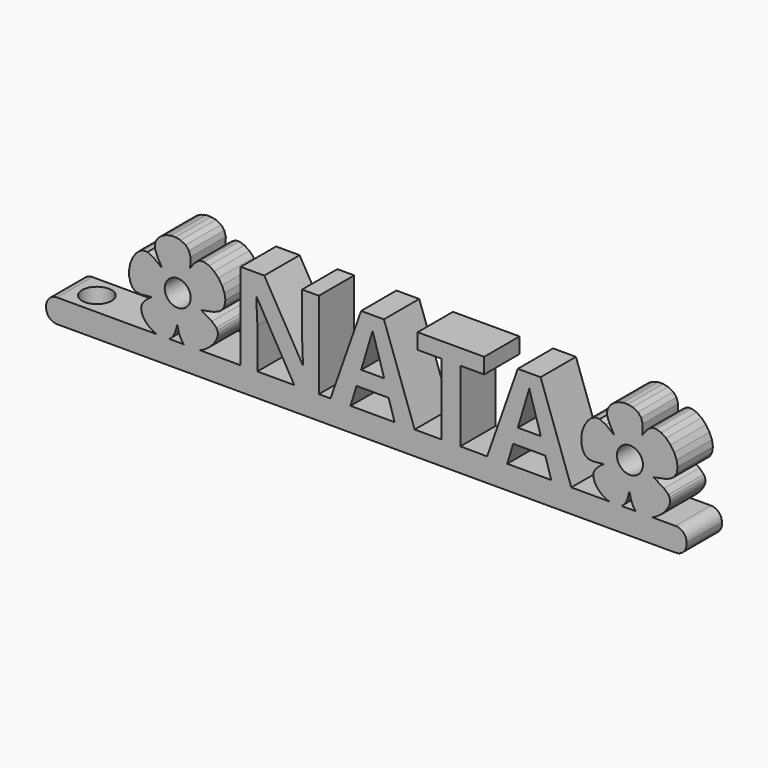
from build123d import *

# Parameters (mm, degrees)
F0_R         = 1.7660260944
F0_TEXT_SIZE = 16.7687842631
F1_DEPTH     = 3
F2_W         = 79.5
F2_H         = 6
F3_DEPTH     = 0.2
F4_DEPTH     = 3
F5_W         = 6
F5_H         = 3.2
F6_DEPTH     = 7.5
F7_R         = 1.5
F8_R         = 2
F9_DEPTH     = 4
F10_R        = 1.5


# Not quite as in the source:
# - Text() gives the source's letters only with a copy of the font that has no kerning and outlines rounded to 1/6400 em; it was checked with that copy


with BuildPart() as f1:
    # F0 (on Front) → F1 (new body, symmetric)
    with BuildSketch(Plane.XZ):
        Polygon((-9.8962181259, -0.0299609487), (-9.3093152472, 0.0995427735), (-8.5310452338, 0.4643787281), (-7.7886221935, 1.0156229815), (-7.1753136859, 1.6703047867), (-6.7844076966, 2.345448762), (-6.6844409889, 2.697736103), (-6.6652413988, 3.0240118702), (-6.7312263226, 3.3305926174), (-6.8868132072, 3.6238062576), (-7.4844896445, 4.1953846804), (-8.4936258745, 4.789299945), (-8.9274018823, 5.0567831788), (-8.4181052429, 5.1580766137), (-7.3131137554, 5.3695361907), (-6.5480905692, 5.6521941874), (-6.0523445823, 6.043851435), (-5.7552051187, 6.5823041299), (-5.6420905942, 7.3346827833), (-5.7751165223, 8.1369112107), (-6.1089634595, 8.9328581362), (-6.5983028952, 9.6663968681), (-7.1978267956, 10.281407439), (-7.8622157172, 10.7217585729), (-8.546147975, 10.9313258196), (-8.8812811082, 10.9320270148), (-9.2043064176, 10.8539824368), (-9.6469000392, 10.5612860557), (-10.1400767255, 9.9810366231), (-10.4508130024, 9.5801644376), (-10.4068223535, 10.0271686751), (-10.3916193646, 10.9311557532), (-10.598433195, 11.6324207168), (-11.0363252865, 12.1480644274), (-11.7143548393, 12.4951945719), (-12.3982545289, 12.6383143795), (-13.0712303381, 12.6247535348), (-13.7032208938, 12.4733707309), (-14.2641853, 12.2030313855), (-14.7240621838, 11.8325941916), (-15.0528129411, 11.3809291004), (-15.2203761991, 10.8668948051), (-15.1967042361, 10.3093544817), (-14.8286469794, 9.4077545862), (-14.3529716358, 8.5454741101), (-14.2906102139, 8.4004774316), (-14.4811582303, 8.5293860258), (-15.3946726039, 9.2300894295), (-16.21802192, 9.6332437342), (-16.8030362894, 9.634121823), (-17.3568401554, 9.3699870508), (-17.8525159958, 8.8932532172), (-18.2631576982, 8.2563454299), (-18.5618432066, 7.5116797807), (-18.7216618753, 6.7116836696), (-18.7156984739, 5.9087754295), (-18.5170445979, 5.1553756349), (-18.2008868091, 4.6439944488), (-17.7512302174, 4.3560670179), (-17.1086136552, 4.2712956407), (-16.2135760559, 4.3694053341), (-15.7044514474, 4.4302814773), (-15.6696932647, 4.4000047008), (-15.7790195709, 4.3290260096), (-16.1651405309, 4.0708069691), (-16.5523139664, 3.7127982689), (-16.8671052824, 3.3322639471), (-17.0360798838, 3.0064680418), (-17.0831036318, 2.6043628391), (-17.0239245605, 2.1921008316), (-16.867618816, 1.7819255621), (-16.6232807801, 1.3860941234), (-16.3000002503, 1.0168545414), (-15.9068693162, 0.6864593752), (-15.4529754831, 0.4071521172), (-14.9474063577, 0.1911989779), (-14.4397479673, 0.0570083052), (-13.9840845603, 0.0188926715), (-13.5797273957, 0.0772799851), (-13.2259605822, 0.2326232662), (-12.9220907946, 0.485341356), (-12.6674066752, 0.8358849825), (-12.4612081239, 1.2846821047), (-12.3027905578, 1.8321743328), (-12.1879723822, 2.2557758958), (-12.1309056827, 2.0998483864), (-12.0112204133, 1.5291342486), (-11.8237778137, 0.9902805659), (-11.5954117235, 0.5466869075), (-11.3529559319, 0.2617414835), (-10.9521058183, 0.053843468), (-10.4551700276, -0.0442881949), align=None)
        with Locations((-12.1185852993, 6.0541479067)):
            Circle(F0_R, mode=Mode.SUBTRACT)
        Polygon((51.2801961291, 9.9810366231), (50.9694598522, 9.5801644376), (51.0134505011, 10.0271686751), (51.02865349, 10.9311557532), (50.8218396596, 11.6324207168), (50.3839475682, 12.1480644274), (49.7059180154, 12.4951945719), (49.0220183257, 12.6383143795), (48.3490425166, 12.6247535348), (47.7170519608, 12.4733707309), (47.1560875547, 12.2030313855), (46.6962106709, 11.8325941916), (46.3674599135, 11.3809291004), (46.1998966555, 10.8668948051), (46.2235686185, 10.3093544817), (46.5916258752, 9.4077545862), (47.0673012188, 8.5454741101), (47.1296626407, 8.4004774316), (46.9391146243, 8.5293860258), (46.0256002507, 9.2300894295), (45.2022509346, 9.6332437342), (44.6172365652, 9.634121823), (44.0634326992, 9.3699870508), (43.5677568588, 8.8932532172), (43.1571151565, 8.2563454299), (42.858429648, 7.5116797807), (42.6986109794, 6.7116836696), (42.7045743808, 5.9087754295), (42.9032282567, 5.1553756349), (43.2193860456, 4.6439944488), (43.6690426372, 4.3560670179), (44.3116591995, 4.2712956407), (45.2066967987, 4.3694053341), (45.7158214073, 4.4302814773), (45.75057959, 4.4000047008), (45.6412532837, 4.3290260096), (45.2551323237, 4.0708069691), (44.8679588882, 3.7127982689), (44.5531675723, 3.3322639471), (44.3841929708, 3.0064680418), (44.3371692228, 2.6043628391), (44.3963482942, 2.1921008316), (44.5526540386, 1.7819255621), (44.7969920745, 1.3860941234), (45.1202726043, 1.0168545414), (45.5134035385, 0.6864593752), (45.9672973716, 0.4071521172), (46.4728664969, 0.1911989779), (46.9805248873, 0.0570083052), (47.4361882943, 0.0188926715), (47.8405454589, 0.0772799851), (48.1943122725, 0.2326232662), (48.49818206, 0.485341356), (48.7528661794, 0.8358849825), (48.9590647307, 1.2846821047), (49.1174822969, 1.8321743328), (49.2323004724, 2.2557758958), (49.2893671719, 2.0998483864), (49.4090524413, 1.5291342486), (49.5964950409, 0.9902805659), (49.8248611311, 0.5466869075), (50.0673169227, 0.2617414835), (50.4681670363, 0.053843468), (50.9651028271, -0.0442881949), (51.5240547287, -0.0299609487), (52.1109576074, 0.0995427735), (52.8892276208, 0.4643787281), (53.6316506611, 1.0156229815), (54.2449591687, 1.6703047867), (54.635865158, 2.345448762), (54.7358318657, 2.697736103), (54.7550314558, 3.0240118702), (54.689046532, 3.3305926174), (54.5334596475, 3.6238062576), (53.9357832101, 4.1953846804), (52.9266469801, 4.789299945), (52.4928709723, 5.0567831788), (53.0021676118, 5.1580766137), (54.1071590993, 5.3695361907), (54.8721822854, 5.6521941874), (55.3679282723, 6.043851435), (55.6650677359, 6.5823041299), (55.7781822604, 7.3346827833), (55.6451563323, 8.1369112107), (55.3113093951, 8.9328581362), (54.8219699594, 9.6663968681), (54.222446059, 10.281407439), (53.5580571374, 10.7217585729), (52.8741248796, 10.9313258196), (52.5389917464, 10.9320270148), (52.2159664371, 10.8539824368), (51.7733728154, 10.5612860557), align=None)
        with Locations((49.3016875553, 6.0541479067)):
            Circle(F0_R, mode=Mode.SUBTRACT)
        with Locations((-5.0709448565, 0)):
            Text('NATA', F0_TEXT_SIZE, font='Open Sans', font_style=FontStyle.BOLD, text_align=(TextAlign.LEFT, TextAlign.BOTTOM))
    extrude(amount=F1_DEPTH, both=True)



with BuildPart() as f3:
    # F2 (on Top) → F3 (new body)
    with BuildSketch(Plane.XY):
        with Locations((17.25, 0)):
            Rectangle(F2_W, F2_H)
    extrude(amount=F3_DEPTH)


with BuildPart() as f4:
    # F4 (new): a face of the model
    f4_faces = [f3.part.faces().sort_by_distance(p)[0] for p in [
        (17.25, 0, 0),
    ]]
    extrude(f4_faces, amount=F4_DEPTH)


with BuildPart() as f1_1:
    add(f1.part)

    add(f3.part)  # F6 merges F3

    add(f4.part)  # F6 merges F4
    # F5 (on face) → F6 (join)
    with BuildSketch(Plane(origin=(-22.5, 0, 0), x_dir=(0, -1, 0), z_dir=(-1, 0, 0))):
        with Locations((0, -1.4)):
            Rectangle(F5_W, F5_H)
    extrude(amount=F6_DEPTH)

    # F7
    f7_edges = [f1_1.edges().sort_by_distance(p)[0] for p in [
        (-30, 0, -3),
        (-30, 0, 0.2),
        (57, 0, -3),
    ]]
    fillet(f7_edges, radius=F7_R)

    # F8 (on face) → F9 (cut)
    with BuildSketch(Plane.XY.offset(0.2)):
        with Locations((-25.5, 0)):
            Circle(F8_R)
    extrude(amount=-F9_DEPTH, mode=Mode.SUBTRACT)

    # F10
    f10_edges = [f1_1.edges().sort_by_distance(p)[0] for p in [
        (57, 0, 0.2),
    ]]
    fillet(f10_edges, radius=F10_R)


solid = f1_1.part
